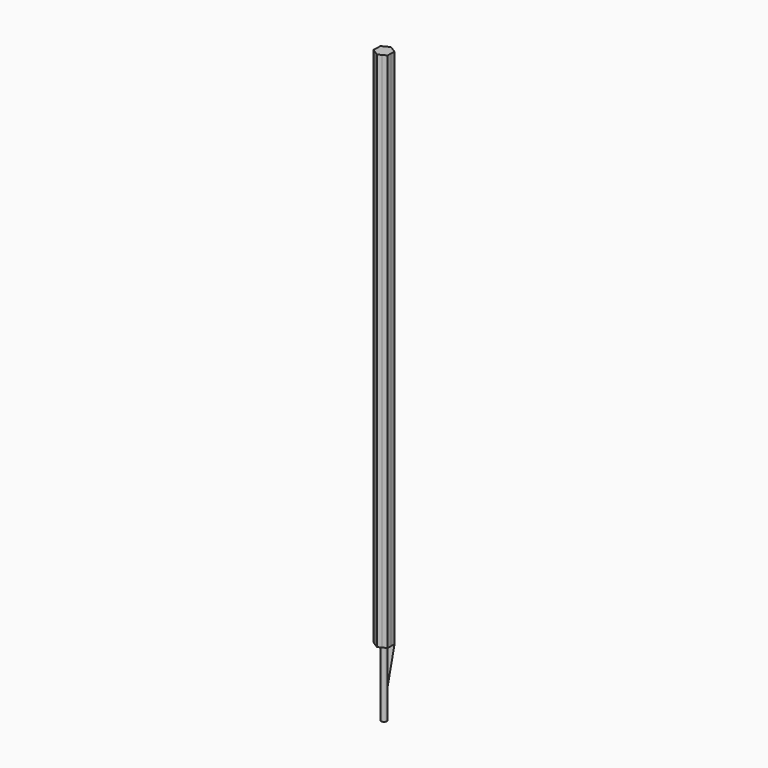
from build123d import *

# Parameters (mm, degrees)
F0_R      = 1
F1_DEPTH  = 180
F2_DEPTH  = 203.3524
F1_FACE_W = 2.8867513459
F1_FACE_H = 180


with BuildPart() as f1:
    # F0 (on Top) → F1 (new body)
    with BuildSketch(Plane.XY):
        with BuildLine():
            ThreePointArc((-1.3365232204, -2.1127483715), (-2.213837243, -1.1614321596), (-2.4979553725, 0.1010888571))
            Line((-2.4979553725, 0.1010888571), (-2.5563190236, -1.3411064025))
            Line((-2.5563190236, -1.3411064025), (-1.3365232204, -2.1127483715))
        make_face()
        with BuildLine():
            Line((-0.1167272981, -2.8843904159), (1.1614322324, -2.2138372048))
            ThreePointArc((1.1614322324, -2.2138372048), (-0.1010888301, -2.4979553736), (-1.3365232204, -2.1127483715))
            Line((-1.3365232204, -2.1127483715), (-0.1167272981, -2.8843904159))
        make_face()
        with BuildLine():
            ThreePointArc((-1.1614322324, 2.2138372048), (0.1010888127, 2.4979553743), (1.3365231909, 2.1127483902))
            Line((1.3365231909, 2.1127483902), (0.1167272981, 2.8843904159))
            Line((0.1167272981, 2.8843904159), (-1.1614322324, 2.2138372048))
        make_face()
        with BuildLine():
            ThreePointArc((-2.4979553725, 0.1010888571), (-2.112748401, 1.3365231738), (-1.1614322324, 2.2138372048))
            Line((-1.1614322324, 2.2138372048), (-2.4395917255, 1.5432840134))
            Line((-2.4395917255, 1.5432840134), (-2.4979553725, 0.1010888571))
        make_face()
        with BuildLine():
            Line((2.4395917255, -1.5432840134), (2.4979553754, -0.101088785))
            ThreePointArc((2.4979553754, -0.101088785), (2.1127484203, -1.3365231433), (1.1614322324, -2.2138372048))
            Line((1.1614322324, -2.2138372048), (2.4395917255, -1.5432840134))
        make_face()
        with BuildLine():
            ThreePointArc((1.3365231909, 2.1127483902), (2.1898981685, 1.2059626907), (2.5, 0))
            ThreePointArc((2.5, 0), (2.4994887916, -0.0505547301), (2.4979553754, -0.101088785))
            Line((2.4979553754, -0.101088785), (2.5563190236, 1.3411064025))
            Line((2.5563190236, 1.3411064025), (1.3365231909, 2.1127483902))
        make_face()
        with BuildLine():
            ThreePointArc((2.4979553754, -0.101088785), (2.4994887916, -0.0505547301), (2.5, 0))
            ThreePointArc((2.5, 0), (2.1898981685, 1.2059626907), (1.3365231909, 2.1127483902))
            ThreePointArc((1.3365231909, 2.1127483902), (0.1010888127, 2.4979553743), (-1.1614322324, 2.2138372048))
            ThreePointArc((-1.1614322324, 2.2138372048), (-2.112748401, 1.3365231738), (-2.4979553725, 0.1010888571))
            ThreePointArc((-2.4979553725, 0.1010888571), (-2.213837243, -1.1614321596), (-1.3365232204, -2.1127483715))
            ThreePointArc((-1.3365232204, -2.1127483715), (-0.1010888301, -2.4979553736), (1.1614322324, -2.2138372048))
            ThreePointArc((1.1614322324, -2.2138372048), (2.1127484203, -1.3365231433), (2.4979553754, -0.101088785))
        make_face()
        Circle(F0_R, mode=Mode.SUBTRACT)
    extrude(amount=-F1_DEPTH)

    # F0 (on Top) → F2 (join)
    with BuildSketch(Plane.XY):
        Circle(F0_R)
    extrude(amount=-F2_DEPTH)

    # F1_face (on face) → F5 section 0
    with BuildSketch(Plane(origin=(1.3365231609, 2.1127484092, -90), x_dir=(-0.8450993637, 0.5346092643, 0), z_dir=(0.5346092643, 0.8450993637, 0)), mode=Mode.PRIVATE) as f5_s0:
        Rectangle(F1_FACE_W, F1_FACE_H)
    loft([Vertex(0, 0, -200), f5_s0.sketch])


solid = f1.part
